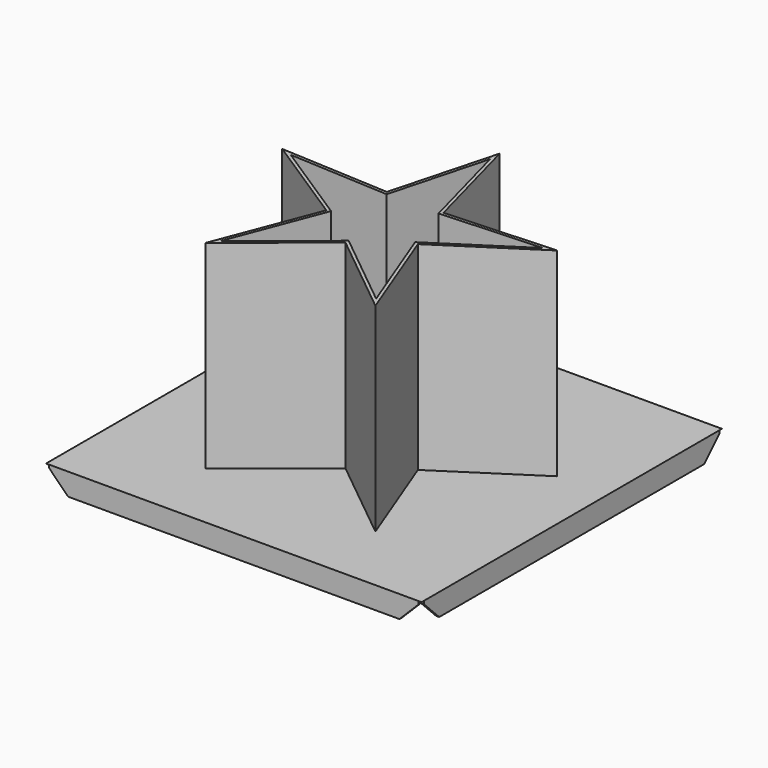
from build123d import *

# Parameters (mm, degrees)
F0_W            = 85
F0_H            = 85
F0_R            = 2
F1_DEPTH        = 0.7
F3_DEPTH        = 45
F4_W            = 85
F4_H            = 85
F4_W_2          = 83.6
F4_H_2          = 83.6
F5_DEPTH        = 4.3
F7_DEPTH        = 25
F7_COPIES_COUNT = 3
F7_COPIES_ANGLE = 180
F9_DEPTH        = 25


# Not quite as in the source:
# - a pattern or mirror of a feature is missing from the dataset's text; its kind, count and spacing are read off the source's solid


with BuildPart() as f1:
    # F0 (on Top) → F1 (new body)
    with BuildSketch(Plane.XY):
        Rectangle(F0_W, F0_H)
        Circle(F0_R, mode=Mode.SUBTRACT)
    extrude(amount=F1_DEPTH)

    # F2 (on face) → F3 (join)
    with BuildSketch(Plane.XY.offset(0.7)):
        Polygon((6.4072893302, 8.8188771933), (0, 32.7312065123), (-6.4072893302, 8.8188771933), (-31.1292272397, 10.1144990587), (-10.367211912, -3.3685113452), (-19.2389204777, -26.4801023149), (0, -10.9007316961), (19.2389204777, -26.4801023149), (10.367211912, -3.3685113452), (31.1292272397, 10.1144990587), align=None)
        Polygon((-5.8778525229, 8.0901699437), (0, 30.0266141987), (5.8778525229, 8.0901699437), (28.557007096, 9.2787340709), (9.510565163, -3.0901699437), (17.6492010023, -24.2920411703), (0, -10), (-17.6492010023, -24.2920411703), (-9.510565163, -3.0901699437), (-28.557007096, 9.2787340709), align=None, mode=Mode.SUBTRACT)
    extrude(amount=F3_DEPTH)

    # F4 (on face) → F5 (join)
    with BuildSketch(Plane(origin=(0, 0, 0), x_dir=(1, 0, 0), z_dir=(0, 0, -1))):
        Rectangle(F4_W, F4_H)
        Rectangle(F4_W_2, F4_H_2, mode=Mode.SUBTRACT)
    extrude(amount=F5_DEPTH)

    # F6 (on face) → F7 (cut)
    with BuildSketch(Plane.YZ.offset(-41.8)):
        Polygon((42.5, -4.3), (42.5, 0.7), (37.5, -4.3), align=None)
        Polygon((-37.5, -4.3), (-42.5, 0.7), (-42.5, -4.3), align=None)
    f7 = extrude(amount=-F7_DEPTH, mode=Mode.SUBTRACT)

    # F7_copies: F7 ×3 about axis
    f7_copies_axis = Axis((0, 0, 0), (0, 0, -1))
    for i in range(1, F7_COPIES_COUNT):
        add(f7.rotate(f7_copies_axis, i * F7_COPIES_ANGLE / (F7_COPIES_COUNT - 1)), mode=Mode.SUBTRACT)

    # F8 (on face) → F9 (cut)
    with BuildSketch(Plane(origin=(0, -41.8, 0), x_dir=(-1, 0, 0), z_dir=(0, 1, 0))):
        Polygon((42.5, -4.3), (42.5, 0.7), (37.5, -4.3), align=None)
        Polygon((-42.5, 0.7), (-42.5, -4.3), (-37.5, -4.3), align=None)
    extrude(amount=-F9_DEPTH, mode=Mode.SUBTRACT)


solid = f1.part
